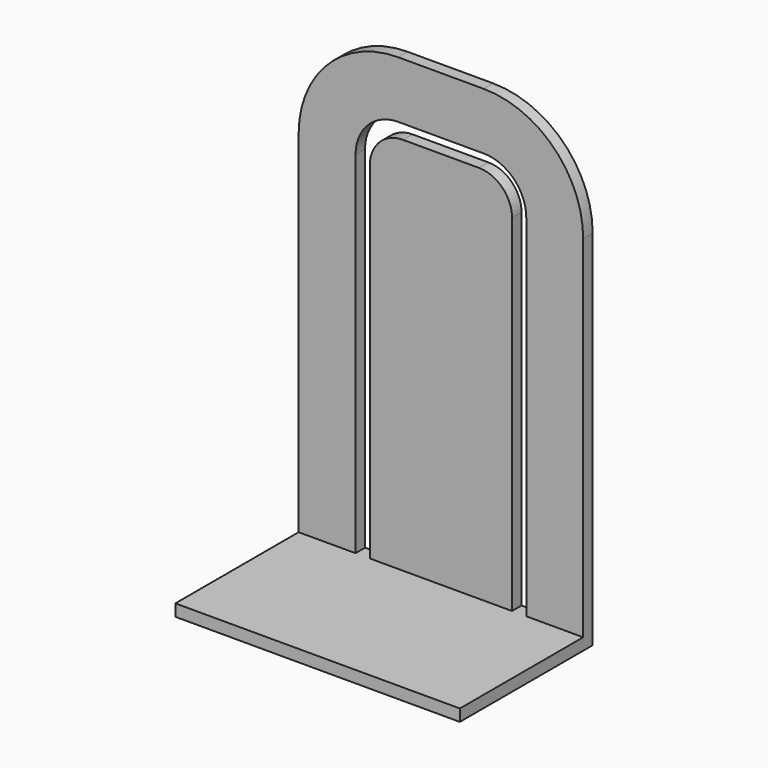
from build123d import *

# Parameters (mm, degrees)
F2_DEPTH = 3.175
F3_W     = 76.2
F3_H     = 44.45
F4_DEPTH = 3.175
F6_DEPTH = 3.175


# Not quite as in the source:
# - a variable given as a bare number and used for a length is read in inches; the dataset says mm whatever the document's units were


with BuildPart() as f2:
    # F1 (on Front) → F2 (new body)
    with BuildSketch(Plane.XZ):
        with BuildLine():
            Line((49.53, 120.65), (26.67, 120.65))
            ThreePointArc((26.67, 120.65), (7.8114621458, 112.8385378542), (0, 93.98))
            Line((0, 93.98), (0, 0))
            Line((0, 0), (15.24, 0))
            Line((15.24, 0), (15.24, 93.98))
            ThreePointArc((15.24, 93.98), (18.587769491, 102.062230509), (26.67, 105.41))
            Line((26.67, 105.41), (49.53, 105.41))
            ThreePointArc((49.53, 105.41), (57.612230509, 102.062230509), (60.96, 93.98))
            Line((60.96, 93.98), (60.96, 0))
            Line((60.96, 0), (76.2, 0))
            Line((76.2, 0), (76.2, 93.98))
            ThreePointArc((76.2, 93.98), (68.3885378542, 112.8385378542), (49.53, 120.65))
        make_face()
    extrude(amount=F2_DEPTH)

    # F3 (on Top) → F4 (join)
    with BuildSketch(Plane.XY):
        with Locations((38.1, -22.225)):
            Rectangle(F3_W, F3_H)
    extrude(amount=-F4_DEPTH)

    # F5 (on Front) → F6 (join)
    with BuildSketch(Plane.XZ):
        with BuildLine():
            Line((48.26, 101.6), (27.94, 101.6))
            ThreePointArc((27.94, 101.6), (21.6538207153, 98.9961792847), (19.05, 92.71))
            Line((19.05, 92.71), (19.05, 0))
            Line((19.05, 0), (57.15, 0))
            Line((57.15, 0), (57.15, 92.71))
            ThreePointArc((57.15, 92.71), (54.5461792847, 98.9961792847), (48.26, 101.6))
        make_face()
    extrude(amount=F6_DEPTH)


solid = f2.part
